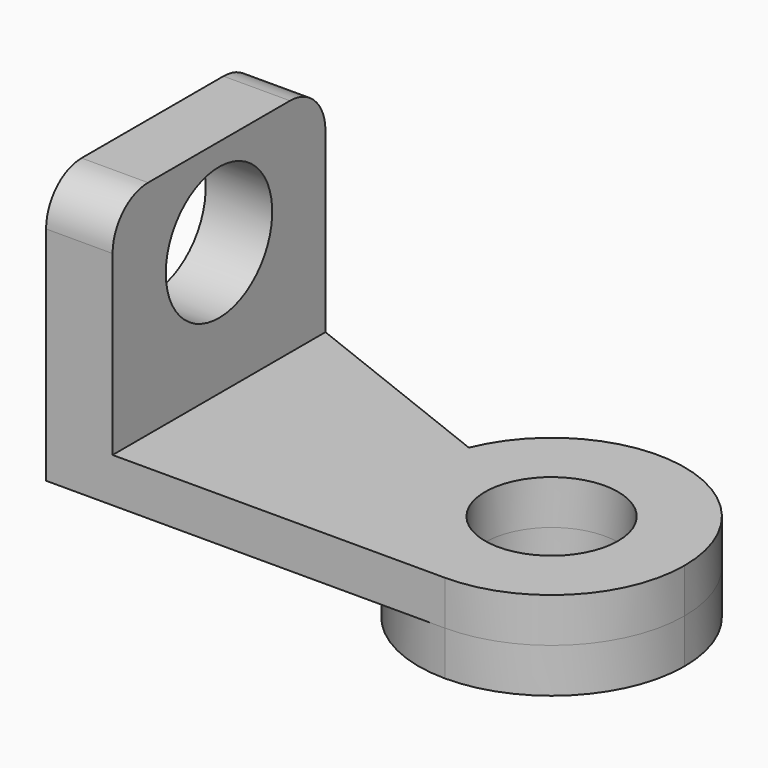
from build123d import *

# Parameters (mm, degrees)
F0_R     = 38.1
F1_DEPTH = 25.4
F2_R     = 38.1
F3_DEPTH = 25.4
F4_R     = 38.1
F5_DEPTH = 38.1


with BuildPart() as f1:
    # F0 (on Top) → F1 (new body)
    with BuildSketch(Plane.XY):
        with BuildLine():
            ThreePointArc((0, -76.2), (53.8815367264, -53.8815367264), (76.2, 0))
            ThreePointArc((76.2, 0), (14.7223801552, 74.7642395973), (-70.5110635844, 28.8899621357))
            ThreePointArc((-70.5110635844, 28.8899621357), (-63.2765956525, -42.4560059665), (0, -76.2))
        make_face()
        Circle(F0_R, mode=Mode.SUBTRACT)
        with BuildLine():
            ThreePointArc((0, -76.2), (-63.2765956525, -42.4560059665), (-70.5110635844, 28.8899621357))
            Line((-70.5110635844, 28.8899621357), (-190.5, 76.2))
            Line((-190.5, 76.2), (-190.5, -76.2))
            Line((-190.5, -76.2), (0, -76.2))
        make_face()
    extrude(amount=F1_DEPTH)

    # F2 (on face) → F3 (join)
    with BuildSketch(Plane(origin=(0, 0, 0), x_dir=(1, 0, 0), z_dir=(0, 0, -1))):
        with BuildLine():
            ThreePointArc((-70.5110635844, -28.8899621357), (14.7223801552, -74.7642395973), (76.2, 0))
            ThreePointArc((76.2, 0), (53.8815367264, 53.8815367264), (0, 76.2))
            ThreePointArc((0, 76.2), (-63.2765956525, 42.4560059665), (-70.5110635844, -28.8899621357))
        make_face()
        Circle(F2_R, mode=Mode.SUBTRACT)
    extrude(amount=F3_DEPTH)

    # F4 (on face) → F5 (join)
    with BuildSketch(Plane(origin=(-190.5, 0, 0), x_dir=(0, -1, 0), z_dir=(-1, 0, 0))):
        with BuildLine():
            Line((-76.2, 0), (76.2, 0))
            Line((76.2, 0), (76.2, 127))
            ThreePointArc((76.2, 127), (68.7605122421, 144.9605122421), (50.8, 152.4))
            Line((50.8, 152.4), (-50.8, 152.4))
            ThreePointArc((-50.8, 152.4), (-68.7605122421, 144.9605122421), (-76.2, 127))
            Line((-76.2, 127), (-76.2, 0))
        make_face()
        with Locations((0, 101.6)):
            Circle(F4_R, mode=Mode.SUBTRACT)
        with BuildLine():
            Line((-76.2, 25.4), (76.2, 25.4))
            Line((76.2, 25.4), (76.2, 127))
            ThreePointArc((76.2, 127), (68.7605122421, 144.9605122421), (50.8, 152.4))
            Line((50.8, 152.4), (-50.8, 152.4))
            ThreePointArc((-50.8, 152.4), (-68.7605122421, 144.9605122421), (-76.2, 127))
            Line((-76.2, 127), (-76.2, 25.4))
        make_face()
        with Locations((0, 101.6)):
            Circle(F4_R, mode=Mode.SUBTRACT)
    extrude(amount=F5_DEPTH)


solid = f1.part
